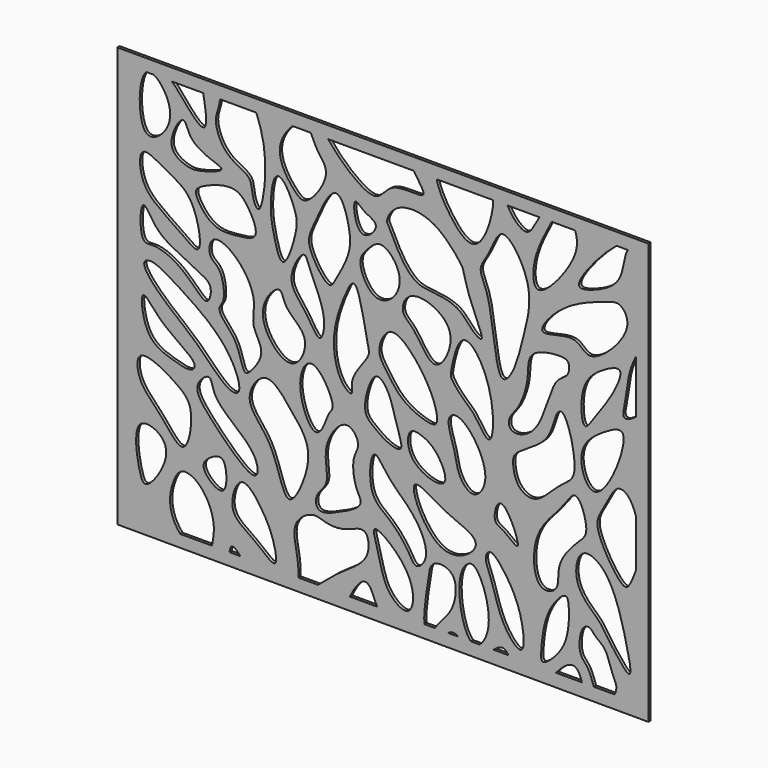
from build123d import *

# Parameters (mm, degrees)
F1_DEPTH = 3


with BuildPart() as f1:
    # F0 (on Front) → F1 (new body)
    with BuildSketch(Plane.XZ):
        with BuildLine():
            add(Edge.make_bspline(
                [(9.7901637022, -246.1338124736), (9.7588059123, -251.7433011661), (9.8231638207, -256.1141962417), (11.7309523035, -257.2440662537)],
                knots=[0.9400744919, 0.9400744919, 0.9400744919, 0.9400744919, 1, 1, 1, 1], degree=3))
            add(Edge.make_bspline(
                [(11.7309523035, -257.2440662537), (14.5146742843, -258.8926997454), (22.0720929935, -252.976389453), (29.3722832782, -246.8268878524), (30.1904138178, -246.1340725422)],
                knots=[0, 0, 0, 0, 0.0874394387, 0.0985039599, 0.0985039599, 0.0985039599, 0.0985039599], degree=3))
            Line((30.1904138178, -246.1340725422), (9.7901637022, -246.1338124736))
        make_face()
        with BuildLine():
            add(Edge.make_bspline(
                [(11.7309523035, -257.2440662537), (14.5146742843, -258.8926997454), (22.0720929935, -252.976389453), (29.3722832782, -246.8268878524), (30.1904138178, -246.1340725422)],
                knots=[0, 0, 0, 0, 0.0874394387, 0.0985039599, 0.0985039599, 0.0985039599, 0.0985039599], degree=3))
            add(Edge.make_bspline(
                [(9.7901637022, -246.1338124736), (9.7588059123, -251.7433011661), (9.8231638207, -256.1141962417), (11.7309523035, -257.2440662537)],
                knots=[0.9400744919, 0.9400744919, 0.9400744919, 0.9400744919, 1, 1, 1, 1], degree=3))
            Line((9.7901637022, -246.1338124736), (-50.3665320084, -246.1330455778))
            add(Edge.make_bspline(
                [(-50.3665320084, -246.1330455778), (-48.3303775027, -248.2458131265), (-43.1270763382, -253.7190469273), (-37.557143271, -257.1762818819), (-34.5870695785, -259.0077182933)],
                knots=[0.0807811304, 0.0807811304, 0.0807811304, 0.0807811304, 0.1240320576, 0.1830256289, 0.1830256289, 0.1830256289, 0.1830256289], degree=3))
            Line((-34.5870695785, -259.0077182933), (58.3993176905, -259.2085698625))
            add(Edge.make_bspline(
                [(63.4588769506, -246.1344966587), (61.4663237301, -250.3922527368), (59.7094369574, -254.9256346001), (58.3993176905, -259.2085698626)],
                knots=[0.6923882564, 0.6923882564, 0.6923882564, 0.6923882564, 0.7375587218, 0.7375587218, 0.7375587218, 0.7375587218], degree=3))
            Line((63.4588769506, -246.1344966587), (30.1904138178, -246.1340725422))
        make_face()
        with BuildLine():
            add(Edge.make_bspline(
                [(30.1904138178, -246.1340725422), (38.4358538211, -239.1516085003), (55.131623573, -224.2446867648), (85.9226539602, -207.4468162091), (81.6135257776, -174.2710504238), (59.1064210203, -188.0247219258), (38.7928820794, -187.8617203747), (24.9584000908, -180.3500590955), (-0.7627512557, -198.2249048598), (10.0492867768, -225.7411908763), (9.8094313103, -242.6870953938), (9.7901637022, -246.1338124736)],
                knots=[0.0985039599, 0.0985039599, 0.0985039599, 0.0985039599, 0.2100165383, 0.3296185811, 0.4228923825, 0.5125673919, 0.6050878351, 0.6821223818, 0.7806699981, 0.9032536186, 0.9400744919, 0.9400744919, 0.9400744919, 0.9400744919], degree=3))
            Line((30.1904138178, -246.1340725422), (63.4588769506, -246.1344966587))
            add(Edge.make_bspline(
                [(91.6403743178, -246.134855925), (88.9294590563, -239.927946458), (83.9082250339, -226.1808906061), (74.3017322339, -227.0352627662), (66.7290897392, -239.1465937843), (63.4588769506, -246.1344966587)],
                knots=[0.4782821954, 0.4782821954, 0.4782821954, 0.4782821954, 0.5486253717, 0.6182537078, 0.6923882564, 0.6923882564, 0.6923882564, 0.6923882564], degree=3))
            Line((91.6403743178, -246.134855925), (140.7887530913, -246.1354824834))
            add(Edge.make_bspline(
                [(150.9457230568, -187.4773949385), (146.6330961136, -190.0849035028), (145.0700738243, -202.6562319311), (141.9604717379, -222.0309323338), (140.3139450852, -237.0479527238), (140.7480163893, -245.5020574078), (140.7887530913, -246.1354824834)],
                knots=[0, 0, 0, 0, 0.1097664917, 0.2358758525, 0.3680330796, 0.378831128, 0.378831128, 0.378831128, 0.378831128], degree=3))
            add(Edge.make_bspline(
                [(151.6535557612, -246.1356209912), (152.0842457989, -245.492729905), (157.8673173196, -237.104152239), (172.5904347604, -225.4697199707), (176.6155565027, -187.0751886755), (155.7266048302, -184.5867692633), (150.9457230568, -187.4773949385)],
                knots=[0.5638155494, 0.5638155494, 0.5638155494, 0.5638155494, 0.575980752, 0.7233184576, 0.8783153223, 1, 1, 1, 1], degree=3))
            Line((151.6535557612, -246.1356209912), (165.5383993688, -246.1357979994))
            add(Edge.make_bspline(
                [(165.5383993688, -246.1357979994), (166.8916685862, -245.1374841957), (168.2456112198, -244.4708527481), (169.5520877838, -244.227617979)],
                knots=[0.9684245262, 0.9684245262, 0.9684245262, 0.9684245262, 1, 1, 1, 1], degree=3))
            add(Edge.make_bspline(
                [(169.5520877838, -244.227617979), (171.7348934141, -243.8212316434), (173.7852007903, -244.5967278838), (175.7411883681, -246.1359280677)],
                knots=[0, 0, 0, 0, 0.0527549624, 0.0527549624, 0.0527549624, 0.0527549624], degree=3))
            Line((175.7411883681, -246.1359280677), (189.226356025, -246.1360999807))
            add(Edge.make_bspline(
                [(185.325473547, -176.8171787262), (182.5084622348, -179.0124112443), (176.5500739638, -188.6532054998), (176.555339328, -219.1069042104), (184.7595727212, -242.227658134), (189.226356025, -246.1360999807)],
                knots=[0, 0, 0, 0, 0.1198377942, 0.3180430449, 0.4608531492, 0.4608531492, 0.4608531492, 0.4608531492], degree=3))
            add(Edge.make_bspline(
                [(198.0807921271, -246.1362128598), (202.4572107284, -242.8113384732), (214.294124997, -220.2269298488), (196.4537099683, -172.0993780413), (187.465245085, -175.1497036822), (185.325473547, -176.8171787262)],
                knots=[0.5460960759, 0.5460960759, 0.5460960759, 0.5460960759, 0.6687120885, 0.9089724986, 1, 1, 1, 1], degree=3))
            Line((198.0807921271, -246.1362128598), (212.7578583264, -246.1363999675))
            add(Edge.make_bspline(
                [(212.7578583264, -246.1363999675), (216.1131583124, -243.0848294513), (219.5559651959, -241.1799456168), (222.2440987825, -241.4247691631)],
                knots=[0.9445554177, 0.9445554177, 0.9445554177, 0.9445554177, 1, 1, 1, 1], degree=3))
            add(Edge.make_bspline(
                [(222.2440987825, -241.4247691631), (224.6132182636, -241.6405382885), (226.3961574475, -243.5260579096), (227.8743273651, -246.1365926768)],
                knots=[0, 0, 0, 0, 0.0488646995, 0.0488646995, 0.0488646995, 0.0488646995], degree=3))
            Line((227.8743273651, -246.1365926768), (277.7129229054, -246.1372280344))
            add(Edge.make_bspline(
                [(277.7129229054, -246.1372280344), (283.6923653133, -238.8513551932), (296.7957777997, -228.067446888), (302.7192229603, -239.3766984719), (304.4872900639, -246.1375693621)],
                knots=[0.3680159099, 0.3680159099, 0.3680159099, 0.3680159099, 0.4564824469, 0.5466627512, 0.5466627512, 0.5466627512, 0.5466627512], degree=3))
            Line((304.4872900639, -246.1375693621), (316.9620559109, -246.1377283942))
            add(Edge.make_bspline(
                [(316.9620559109, -246.1377283942), (315.1592613006, -240.7444351763), (310.8096705188, -228.164972779), (300.0346077167, -222.3203557149), (302.9818520324, -194.8007969424), (310.2238803249, -192.6842301325), (312.23320961, -193.430557847)],
                knots=[0.6529297592, 0.6529297592, 0.6529297592, 0.6529297592, 0.7271660182, 0.8177156532, 0.9357279799, 1, 1, 1, 1], degree=3))
            add(Edge.make_bspline(
                [(312.23320961, -193.430557847), (314.3987465407, -194.2349059647), (317.9201942459, -200.0632035933), (330.6257744805, -206.8171760044), (334.6111704969, -227.0036269584), (341.6905925863, -237.1679193511), (339.7554115606, -243.7170809246), (338.6080290375, -246.1380043437)],
                knots=[0, 0, 0, 0, 0.0692686033, 0.1590658267, 0.2671580117, 0.3555247119, 0.4051353819, 0.4051353819, 0.4051353819, 0.4051353819], degree=3))
            Line((338.6080290375, -246.1380043437), (360.9821200371, -246.1382895754))
            Line((360.9821200371, -246.1382895754), (360.9821200371, -124.6424126949))
            add(Edge.make_bspline(
                [(342.0082628727, -56.7098855972), (337.8376569664, -58.6143161112), (331.7078660667, -71.4640421648), (322.8482168883, -85.7041512548), (316.6274138765, -102.0127331196), (347.5547979066, -150.7207499406), (354.6205927365, -140.2264698905), (359.0749163627, -130.6088737094), (360.9821200371, -124.6424126949)],
                knots=[0, 0, 0, 0, 0.1084019294, 0.2154866103, 0.3238733132, 0.5061092667, 0.5780773791, 0.6571797703, 0.6571797703, 0.6571797703, 0.6571797703], degree=3))
            add(Edge.make_bspline(
                [(360.9821200371, -76.531337101), (359.0514846438, -70.245651789), (353.2660580691, -58.0597419764), (345.5294972833, -55.1019786386), (342.0082628727, -56.7098855972)],
                knots=[0.8351803062, 0.8351803062, 0.8351803062, 0.8351803062, 0.908476463, 1, 1, 1, 1], degree=3))
            Line((360.9821200371, -76.531337101), (360.9821200371, 15.1898744979))
            add(Edge.make_bspline(
                [(360.9821200371, 15.1898744979), (355.6565059721, 11.1423212631), (350.6052370501, 8.7464678831), (348.6705720425, 10.5318771675)],
                knots=[0.8984641801, 0.8984641801, 0.8984641801, 0.8984641801, 1, 1, 1, 1], degree=3))
            add(Edge.make_bspline(
                [(348.6705720425, 10.5318771675), (346.1789182244, 12.8313046357), (352.3475964652, 34.1049078926), (352.0242052067, 51.6807917861), (359.6520995719, 68.2783470175), (360.9821200371, 70.9079119016)],
                knots=[0, 0, 0, 0, 0.1307679171, 0.3012406905, 0.3329604649, 0.3329604649, 0.3329604649, 0.3329604649], degree=3))
            Line((360.9821200371, 70.9079119016), (360.9821200371, 165.1975970457))
            Line((360.9821200371, 165.1975970457), (352.5482071967, 165.1975970457))
            add(Edge.make_bspline(
                [(352.4027168751, 164.9963259697), (352.4506544554, 165.0640860413), (352.4991627821, 165.131172959), (352.5482071967, 165.1975970457)],
                knots=[0.5045050801, 0.5045050801, 0.5045050801, 0.5045050801, 0.5064013288, 0.5064013288, 0.5064013288, 0.5064013288], degree=3))
            add(Edge.make_bspline(
                [(301.554620266, 116.592861712), (301.9530032289, 112.4990153253), (320.233240766, 117.1712219456), (349.144625433, 132.3748423439), (347.8079865703, 158.5016457505), (352.4027168751, 164.9963259697)],
                knots=[0, 0, 0, 0, 0.1299762549, 0.3227530746, 0.5045050801, 0.5045050801, 0.5045050801, 0.5045050801], degree=3))
            add(Edge.make_bspline(
                [(340.6141401268, 165.1975970457), (323.4581870006, 151.6388907619), (300.8248964657, 124.0916189903), (301.554620266, 116.592861712)],
                knots=[0.7619206254, 0.7619206254, 0.7619206254, 0.7619206254, 1, 1, 1, 1], degree=3))
            Line((340.6141401268, 165.1975970457), (316.197607198, 165.1975970457))
            add(Edge.make_bspline(
                [(312.9373053891, 165.1975970457), (313.7379383521, 164.6227509115), (314.7385961218, 164.5574802886), (316.0388133955, 165.1217950158), (316.197607198, 165.1975970457)],
                knots=[0.3221219636, 0.3221219636, 0.3221219636, 0.3221219636, 0.3594895273, 0.3645407278, 0.3645407278, 0.3645407278, 0.3645407278], degree=3))
            Line((312.9373053891, 165.1975970457), (297.5711116065, 165.1975970457))
            add(Edge.make_bspline(
                [(297.5711116065, 165.1975970457), (299.4289483797, 159.056886812), (303.0083586173, 140.1668971596), (268.7535906867, 98.0109773184), (259.5071792603, 98.5026732087)],
                knots=[0.6614479245, 0.6614479245, 0.6614479245, 0.6614479245, 0.7737000347, 1, 1, 1, 1], degree=3))
            add(Edge.make_bspline(
                [(259.5071792603, 98.5026732087), (254.0550463277, 98.7926009691), (252.3186900207, 124.0218742831), (263.2709078544, 146.1532628497), (272.1856793908, 163.3292534028), (273.1705281061, 165.1975970457)],
                knots=[0, 0, 0, 0, 0.1334374425, 0.3281816369, 0.3520603533, 0.3520603533, 0.3520603533, 0.3520603533], degree=3))
            Line((273.1705281061, 165.1975970457), (260.5168320192, 165.1975970457))
            add(Edge.make_bspline(
                [(245.8173036575, 147.3950594664), (250.5583563735, 147.0523913273), (253.9924391368, 154.4900621523), (259.1169298408, 162.9643350938), (260.5168320192, 165.1975970457)],
                knots=[0, 0, 0, 0, 0.0827283575, 0.1116799116, 0.1116799116, 0.1116799116, 0.1116799116], degree=3))
            add(Edge.make_bspline(
                [(227.3503893477, 165.1975970457), (231.4225669247, 156.4975025172), (240.1755924408, 147.8028243236), (245.8173036575, 147.3950594664)],
                knots=[0.9015557239, 0.9015557239, 0.9015557239, 0.9015557239, 1, 1, 1, 1], degree=3))
            Line((227.3503893477, 165.1975970457), (212.3341254649, 165.1975970457))
            add(Edge.make_bspline(
                [(155.0230979919, 160.0361615419), (156.8732559449, 154.6766413761), (163.0714439049, 142.2896208272), (181.5890181301, 117.4369562013), (199.8519668676, 117.5588360405), (210.5976716303, 145.8389913841), (212.3245910057, 161.3691844962), (212.3341254649, 165.1975970457)],
                knots=[0, 0, 0, 0, 0.1072129517, 0.2385789935, 0.3255263098, 0.4690536374, 0.5179348553, 0.5179348553, 0.5179348553, 0.5179348553], degree=3))
            add(Edge.make_bspline(
                [(153.6499642193, 165.1975970457), (153.940582741, 163.4251992855), (154.4345182879, 161.7411536958), (155.0230979919, 160.0361615419)],
                knots=[0.9658929837, 0.9658929837, 0.9658929837, 0.9658929837, 1, 1, 1, 1], degree=3))
            Line((153.6499642193, 165.1975970457), (129.826022755, 165.1975970457))
            add(Edge.make_bspline(
                [(91.6477292776, 129.5943558216), (97.3979884485, 131.7922597709), (105.2485675897, 149.8823023767), (147.9146265598, 140.6352041492), (135.593177157, 155.9927611171), (130.8858030033, 163.4806066542), (129.826022755, 165.1975970457)],
                knots=[0, 0, 0, 0, 0.0856459715, 0.1836942568, 0.253366065, 0.274225406, 0.274225406, 0.274225406, 0.274225406], degree=3))
            add(Edge.make_bspline(
                [(40.8015214916, 165.1975970457), (49.0526624832, 154.4726750808), (67.6534973731, 136.8247102001), (85.8715274154, 127.3865358769), (91.6477292776, 129.5943558216)],
                knots=[0.8012274033, 0.8012274033, 0.8012274033, 0.8012274033, 0.9139676307, 1, 1, 1, 1], degree=3))
            Line((40.8015214916, 165.1975970457), (22.6455849149, 165.1975970457))
            add(Edge.make_bspline(
                [(22.6455849149, 165.1975970457), (24.6398958382, 161.6370109703), (29.5538657027, 148.2355516574), (47.0601388111, 135.1221054363), (18.7166898876, 95.5205719357), (5.0069116738, 106.1424772606), (-17.6160930997, 136.0140279301), (-2.2030845369, 159.677612741), (3.8405073166, 165.1975970457)],
                knots=[0.0698097678, 0.0698097678, 0.0698097678, 0.0698097678, 0.1481908, 0.2995346732, 0.4930544209, 0.6052153218, 0.8046207697, 0.9189939387, 0.9189939387, 0.9189939387, 0.9189939387], degree=3))
            Line((3.8405073166, 165.1975970457), (-34.0658859726, 165.1975970457))
            add(Edge.make_bspline(
                [(-71.6462448819, 165.1975970457), (-72.2969683467, 157.3510943413), (-79.7183107043, 145.6816655054), (-68.6377171634, 119.6547763879), (-53.3257447767, 110.2585347544), (-38.2399788393, 103.6005996281), (-38.614635353, 86.7659803961), (-31.1317027167, 72.1252851471), (-24.62202919, 96.8150655062), (-23.2706553709, 134.0637171072), (-30.9532538043, 157.4744689897), (-34.0658859726, 165.1975970457)],
                knots=[0.089928055, 0.089928055, 0.089928055, 0.089928055, 0.1676987467, 0.2527597183, 0.3254280955, 0.3898837418, 0.4591848219, 0.5122515839, 0.581435558, 0.6977227887, 0.7653792045, 0.7653792045, 0.7653792045, 0.7653792045], degree=3))
            Line((-71.6462448819, 165.1975970457), (-89.0812227176, 165.1975970457))
            add(Edge.make_bspline(
                [(-89.0812227176, 165.1975970457), (-86.8017226668, 153.5122763774), (-81.940175123, 120.319503587), (-107.9165107445, 149.4971925596), (-117.6975816285, 161.9199339716), (-121.8640712604, 165.1975970457)],
                knots=[0.3704020456, 0.3704020456, 0.3704020456, 0.3704020456, 0.4942900576, 0.6199661345, 0.6995310505, 0.6995310505, 0.6995310505, 0.6995310505], degree=3))
            Line((-121.8640712604, 165.1975970457), (-140.5946574464, 165.1975970457))
            add(Edge.make_bspline(
                [(-140.5946574464, 165.1975970457), (-134.9257063203, 162.2886488757), (-119.4787882332, 141.7502735529), (-125.928966429, 114.6992790111), (-144.2378376817, 104.6267474873), (-149.1714119911, 110.2871596813)],
                knots=[0.401597112, 0.401597112, 0.401597112, 0.401597112, 0.5621504349, 0.8086075159, 1, 1, 1, 1], degree=3))
            add(Edge.make_bspline(
                [(-149.1714119911, 110.2871596813), (-157.5416921129, 119.8905897092), (-157.0763635952, 158.4606170832), (-148.0610253078, 165.1975970457)],
                knots=[0, 0, 0, 0, 0.324715633, 0.324715633, 0.324715633, 0.324715633], degree=3))
            Line((-148.0610253078, 165.1975970457), (-165.7420098782, 165.1975970457))
            Line((-165.7420098782, 165.1975970457), (-165.7420098782, -246.1382895754))
            Line((-165.7420098782, -246.1382895754), (-113.0190528962, -246.1382895754))
            add(Edge.make_bspline(
                [(-111.2022027373, -188.2839649916), (-115.7367334985, -190.1385830578), (-121.4688091599, -202.2879183309), (-125.0870479005, -219.505637695), (-121.1606821222, -235.3049207758), (-114.6758142992, -244.1395123904), (-113.0190528962, -246.1382895754)],
                knots=[0, 0, 0, 0, 0.0923866418, 0.1889201522, 0.2950886497, 0.3264831601, 0.3264831601, 0.3264831601, 0.3264831601], degree=3))
            add(Edge.make_bspline(
                [(-79.9855316672, -246.1326679858), (-78.979360547, -240.8248467781), (-75.4830066636, -221.8614278802), (-89.7581656824, -192.8295221067), (-106.360277204, -186.3036228035), (-111.2022027373, -188.2839649916)],
                knots=[0.7014049055, 0.7014049055, 0.7014049055, 0.7014049055, 0.7597148887, 0.9013504895, 1, 1, 1, 1], degree=3))
            Line((-79.9855316672, -246.1326679858), (-61.7217507226, -246.132900818))
            add(Edge.make_bspline(
                [(-61.7217507226, -246.132900818), (-61.3553102235, -242.982915953), (-60.5950676776, -240.7594567784), (-59.4025216997, -240.0836497545)],
                knots=[0.9519600349, 0.9519600349, 0.9519600349, 0.9519600349, 1, 1, 1, 1], degree=3))
            add(Edge.make_bspline(
                [(-59.4025216997, -240.0836497545), (-57.397207753, -238.9472531079), (-54.1695224407, -242.186962532), (-50.3665320084, -246.1330455778)],
                knots=[0, 0, 0, 0, 0.0807811304, 0.0807811304, 0.0807811304, 0.0807811304], degree=3))
            Line((-50.3665320084, -246.1330455778), (9.7901637022, -246.1338124736))
        make_face()
        with BuildLine():
            add(Edge.make_bspline(
                [(-49.0425825119, -177.9240220785), (-42.8470364952, -175.9658380857), (-26.747837749, -196.6289989175), (-15.6036590183, -218.4973309131), (-10.2543517306, -250.6961493178), (-37.5967274964, -223.2187291122), (-65.5230366459, -210.84902308), (-55.5631052255, -179.9849192405), (-49.0425825119, -177.9240220785)],
                knots=[0, 0, 0, 0, 0.163821842, 0.3437585205, 0.4833218477, 0.6484554387, 0.8275851654, 1, 1, 1, 1], degree=3))
        make_face(mode=Mode.SUBTRACT)
        with BuildLine():
            add(Edge.make_bspline(
                [(-154.7139436007, -159.2761427164), (-162.0673137426, -166.5822235647), (-156.2899293947, -203.4468910848), (-148.775531084, -218.1461415178), (-125.5891043797, -187.0420821525), (-127.5237587016, -161.4356635882), (-149.5291516341, -154.124693985), (-154.7139436007, -159.2761427164)],
                knots=[0, 0, 0, 0, 0.2661661973, 0.3945228903, 0.6168433641, 0.8123287235, 1, 1, 1, 1], degree=3))
        make_face(mode=Mode.SUBTRACT)
        with BuildLine():
            add(Edge.make_bspline(
                [(-154.7139436007, -117.8363934159), (-150.3330004414, -128.1604054443), (-133.7235727782, -140.5181794193), (-107.025270693, -181.4076993717), (-97.9114632331, -127.5386921075), (-112.5996499207, -110.9999080575), (-160.1993723872, -84.4868963537), (-158.1885838415, -109.6481503056), (-154.7139436007, -117.8363934159)],
                knots=[0, 0, 0, 0, 0.1762482162, 0.3424839636, 0.5175769137, 0.6707372224, 0.8602129445, 1, 1, 1, 1], degree=3))
        make_face(mode=Mode.SUBTRACT)
        with BuildLine():
            add(Edge.make_bspline(
                [(-83.1116363406, -167.107462883), (-86.8950146982, -170.0166810192), (-94.1015318841, -178.4470759392), (-64.2507972163, -203.6432671878), (-64.3495703263, -169.2194988193), (-70.9241249433, -160.0006980719), (-79.3594135294, -164.2222017165), (-83.1116363406, -167.107462883)],
                knots=[0, 0, 0, 0, 0.1793282299, 0.4240380764, 0.6648174361, 0.8221485109, 1, 1, 1, 1], degree=3))
        make_face(mode=Mode.SUBTRACT)
        with BuildLine():
            add(Edge.make_bspline(
                [(-94.6263149381, -103.3324822783), (-97.3351273693, -111.3066536379), (-82.1513836519, -130.6274937722), (-30.5261311673, -182.3501636577), (-32.2249762364, -141.5247921608), (-80.830203768, -114.8528230357), (-79.6288248503, -86.5475214013), (-92.7324826989, -97.7574403792), (-94.6263149381, -103.3324822783)],
                knots=[0, 0, 0, 0, 0.1696352952, 0.3986729263, 0.5292755047, 0.7562551812, 0.8814016108, 1, 1, 1, 1], degree=3))
        make_face(mode=Mode.SUBTRACT)
        with BuildLine():
            add(Edge.make_bspline(
                [(-151.437535882, -40.0536358356), (-149.2210512947, -38.4603234546), (-137.7795959471, -54.3524178919), (-118.0480813781, -69.3715854838), (-94.7919748909, -84.598481614), (-101.4264509751, -94.8120633896), (-122.7162799821, -88.8718402019), (-150.44874113, -79.5390002198), (-154.5821508584, -42.3141315793), (-151.437535882, -40.0536358356)],
                knots=[0, 0, 0, 0, 0.1233388014, 0.2925025537, 0.4419871436, 0.5200136835, 0.6563686945, 0.8250143294, 1, 1, 1, 1], degree=3))
        make_face(mode=Mode.SUBTRACT)
        with BuildLine():
            add(Edge.make_bspline(
                [(-150.5026966333, -11.0736070201), (-150.4893487051, -17.3355469245), (-126.2152665406, -42.6351071505), (-94.7569613857, -64.5684509849), (-65.3041487641, -99.3539826394), (-46.6543602503, -98.6276226274), (-62.6024893437, -54.8362913711), (-110.5945621284, -22.9231924262), (-143.0495610241, -2.8415781502), (-150.5087707517, -8.224043874), (-150.5026966333, -11.0736070201)],
                knots=[0, 0, 0, 0, 0.1322321478, 0.2823248202, 0.4289628952, 0.4972210274, 0.6304299889, 0.8086347478, 0.939826338, 1, 1, 1, 1], degree=3))
        make_face(mode=Mode.SUBTRACT)
        with BuildLine():
            add(Edge.make_bspline(
                [(0, -177.4109601974), (5.8200221993, -178.1370236931), (21.2026976084, -145.2132493719), (20.6495023203, -117.3443166746), (1.0015963147, -94.1253142853), (-24.1127550851, -63.1248739152), (-51.1629892185, -103.5894306607), (-14.293252374, -127.6052780443), (-6.8005060178, -176.5625786961), (0, -177.4109601974)],
                knots=[0, 0, 0, 0, 0.1427258357, 0.2751074907, 0.4104542502, 0.5445432786, 0.675497511, 0.8332295185, 1, 1, 1, 1], degree=3))
        make_face(mode=Mode.SUBTRACT)
        with BuildLine():
            add(Edge.make_bspline(
                [(29.0527436882, -165.0769263506), (31.2395066331, -159.5630187032), (44.9159701153, -150.1849526604), (31.4570289031, -118.0637373663), (59.2891467403, -79.8804512916), (75.8000423543, -104.7237414977), (64.7835769051, -116.4842560456), (67.9701329048, -144.8221419535), (79.7959889027, -159.1493961431), (53.5033760291, -172.0515429332), (28.835559846, -182.3442693433), (27.2907319165, -169.5198268512), (29.0527436882, -165.0769263506)],
                knots=[0, 0, 0, 0, 0.0933625362, 0.2163559826, 0.3440104059, 0.4348205419, 0.5177258055, 0.6310963589, 0.7117318364, 0.821188626, 0.9247719611, 1, 1, 1, 1], degree=3))
        make_face(mode=Mode.SUBTRACT)
        with BuildLine():
            add(Edge.make_bspline(
                [(24.7797649354, -46.1300946772), (33.4841423853, -48.1610374633), (49.9295556285, -77.7408917815), (41.0382183293, -84.223270109), (37.2344758871, -98.5719609378), (25.0455020105, -115.9992902392), (4.5933329876, -68.737967041), (17.5128248481, -44.4345409593), (24.7797649354, -46.1300946772)],
                knots=[0, 0, 0, 0, 0.216780114, 0.3243111701, 0.4642219083, 0.5877696991, 0.8190188661, 1, 1, 1, 1], degree=3))
        make_face(mode=Mode.SUBTRACT)
        with BuildLine():
            add(Edge.make_bspline(
                [(80.4027318954, -74.1752907634), (82.0467210946, -78.0943267376), (89.229057935, -83.1695231565), (100.5726733877, -92.4164954968), (121.2433396864, -98.0621788598), (111.0017186855, -72.9307433961), (106.2914892853, -47.8955258557), (90.5010452837, -28.504632203), (79.7990264357, -53.3568625242), (78.2222110363, -68.9772397701), (80.4027318954, -74.1752907634)],
                knots=[0, 0, 0, 0, 0.102251427, 0.2199368704, 0.3280782412, 0.4554437385, 0.6155828309, 0.7332437765, 0.8643778381, 1, 1, 1, 1], degree=3))
        make_face(mode=Mode.SUBTRACT)
        with BuildLine():
            add(Edge.make_bspline(
                [(89.410841465, -175.7564544678), (86.6030560203, -177.2233677412), (94.366061844, -197.815945156), (98.8409064083, -228.734502778), (123.7839973339, -245.6969403956), (131.9750770063, -225.5342598057), (121.9674910588, -195.3771845413), (93.1158460088, -173.8207936239), (89.410841465, -175.7564544678)],
                knots=[0, 0, 0, 0, 0.1442767921, 0.3405895945, 0.4935831484, 0.6164220744, 0.809620008, 1, 1, 1, 1], degree=3))
        make_face(mode=Mode.SUBTRACT)
        with BuildLine():
            add(Edge.make_bspline(
                [(204.7077417374, -163.8956665993), (204.1523225453, -168.6485935078), (211.6683604624, -182.3062631169), (219.8238730584, -220.7434793935), (247.1471601877, -247.7798983258), (242.2585468756, -201.0883152829), (226.7729628555, -174.0459785633), (209.8460474977, -153.4490082691), (205.0653686655, -160.8353210545), (204.7077417374, -163.8956665993)],
                knots=[0, 0, 0, 0, 0.1236765591, 0.3143041835, 0.4507721866, 0.6117599636, 0.7901366256, 0.9203663313, 1, 1, 1, 1], degree=3))
        make_face(mode=Mode.SUBTRACT)
        with BuildLine():
            add(Edge.make_bspline(
                [(263.7775242329, -240.5017912388), (266.2082045074, -241.3172040158), (278.8113733746, -230.5387872285), (291.0252753674, -211.4965624071), (291.8551974369, -179.5938069576), (287.5889582541, -168.4423483181), (266.3406562061, -191.4777978965), (262.3643964417, -225.5266234953), (261.613343229, -239.775780146), (263.7775242329, -240.5017912388)],
                knots=[0, 0, 0, 0, 0.1230988977, 0.2820872387, 0.4589053959, 0.5387575037, 0.6938434852, 0.8903976394, 1, 1, 1, 1], degree=3))
        make_face(mode=Mode.SUBTRACT)
        with BuildLine():
            add(Edge.make_bspline(
                [(88.678278029, -107.6285466552), (91.9390645239, -105.9309566943), (103.37699785, -127.335172652), (131.0999306085, -147.0863165568), (148.3542447523, -183.2261837364), (131.5732441289, -200.1687303011), (124.5569320843, -184.0548745939), (105.564771734, -160.4088417201), (81.2425974722, -148.3974638869), (84.4177193629, -109.8466255238), (88.678278029, -107.6285466552)],
                knots=[0, 0, 0, 0, 0.1102741842, 0.2642143755, 0.411244528, 0.504785479, 0.5914271891, 0.7272813755, 0.8559152426, 1, 1, 1, 1], degree=3))
        make_face(mode=Mode.SUBTRACT)
        with BuildLine():
            add(Edge.make_bspline(
                [(130.4340958595, -122.2797185183), (133.0400681692, -117.8271601762), (154.9141954368, -132.3650170442), (174.6052962396, -141.4299827917), (184.8133512468, -144.7470659296), (203.4744474996, -157.4013365851), (154.8156762099, -192.0919576276), (126.3803245372, -129.2059829497), (130.4340958595, -122.2797185183)],
                knots=[0, 0, 0, 0, 0.1600323205, 0.3226553408, 0.4319117618, 0.5546081218, 0.7510585861, 1, 1, 1, 1], degree=3))
        make_face(mode=Mode.SUBTRACT)
        with BuildLine():
            add(Edge.make_bspline(
                [(214.1752690077, -126.3125836849), (213.0041878255, -120.7514142857), (219.8665971717, -92.0211380051), (247.2077011259, -156.7016947172), (223.3830926025, -131.5769554034), (215.1725210623, -131.0482823655), (214.1752690077, -126.3125836849)],
                knots=[0, 0, 0, 0, 0.2354488004, 0.5758462886, 0.7994999804, 1, 1, 1, 1], degree=3))
        make_face(mode=Mode.SUBTRACT)
        with BuildLine():
            add(Edge.make_bspline(
                [(126.4401078224, -74.6891573071), (122.5239643988, -78.7963365946), (122.1914860804, -105.5016182127), (171.8867005439, -120.2022014193), (154.5217244599, -82.3185468825), (138.6629526756, -74.0680619172), (128.9665956425, -72.0394232902), (126.4401078224, -74.6891573071)],
                knots=[0, 0, 0, 0, 0.2145358952, 0.4572378776, 0.6719930307, 0.8615928306, 1, 1, 1, 1], degree=3))
        make_face(mode=Mode.SUBTRACT)
        with BuildLine():
            add(Edge.make_bspline(
                [(166.3480997086, -50.0724948943), (165.339349991, -53.8293485495), (167.8059829942, -64.5023735653), (172.8796792164, -77.7862206967), (175.1067187168, -98.9759395974), (192.7650047576, -117.4716066646), (211.7732201054, -90.28459381), (188.8626985545, -50.1715455029), (171.8555726807, -42.495848002), (167.0896117461, -47.3109058102), (166.3480997086, -50.0724948943)],
                knots=[0, 0, 0, 0, 0.1072274123, 0.2184521607, 0.3534504855, 0.4775216841, 0.6138949518, 0.806442624, 0.9211792424, 1, 1, 1, 1], degree=3))
        make_face(mode=Mode.SUBTRACT)
        with BuildLine():
            add(Edge.make_bspline(
                [(298.4280288219, -77.6777416468), (294.3040478163, -76.2921197484), (285.3245136432, -92.9330899627), (266.9607307519, -109.5939483237), (254.2974671212, -132.5074819859), (253.9787997513, -162.4284662391), (264.0055531453, -177.0898088384), (282.7198889127, -169.7764116334), (276.3853521731, -144.0342812686), (301.8707693717, -117.4401451098), (313.0906701859, -107.3213697907), (303.6815574574, -79.4428817652), (298.4280288219, -77.6777416468)],
                knots=[0, 0, 0, 0, 0.089039436, 0.1991282231, 0.3063955203, 0.4206241499, 0.5006279828, 0.5781437498, 0.679347374, 0.8034575627, 0.8865728949, 1, 1, 1, 1], degree=3))
        make_face(mode=Mode.SUBTRACT)
        with BuildLine():
            add(Edge.make_bspline(
                [(320.2433586121, -182.1674406528), (315.0293316685, -177.2312605891), (294.1076481921, -160.5979135941), (301.2426859067, -119.5148667501), (335.3720060402, -135.3617989296), (350.0969142683, -190.8118410895), (360.1255769026, -238.3022753521), (326.6233242913, -190.0170173632), (323.5883525267, -185.3341853692), (320.2433586121, -182.1674406528)],
                knots=[0, 0, 0, 0, 0.1448937229, 0.2850223124, 0.4100184393, 0.6163278528, 0.7466596125, 0.9070452403, 1, 1, 1, 1], degree=3))
        make_face(mode=Mode.SUBTRACT)
        with BuildLine():
            add(Edge.make_bspline(
                [(236.7578595877, -58.3544187248), (233.4174400822, -61.5484116014), (232.2154075405, -68.4015899654), (236.0209966684, -89.5785470863), (257.8189356159, -99.9048926577), (279.7234921928, -72.2889373982), (300.9871564905, -62.6496735389), (294.0883347349, -29.2864091892), (292.9212875683, -23.6663982251), (285.4334244258, -1.6793656627), (275.5688921703, -10.0688717682), (272.9732415071, -39.5210960893), (243.000607579, -52.3853203579), (236.7578595877, -58.3544187248)],
                knots=[0, 0, 0, 0, 0.067514333, 0.1583364668, 0.2452279255, 0.3606221189, 0.4560086657, 0.5648975457, 0.6243667374, 0.7119562791, 0.7653898758, 0.8738257378, 1, 1, 1, 1], degree=3))
        make_face(mode=Mode.SUBTRACT)
        with BuildLine():
            add(Edge.make_bspline(
                [(347.3724424839, -5.4615912959), (345.2195292571, 0.3874205669), (324.6361905848, -10.2574458769), (295.0940784516, -32.7534033867), (320.6048718538, -95.3127561624), (351.3976862076, -16.3973308311), (347.3724424839, -5.4615912959)],
                knots=[0, 0, 0, 0, 0.1796549949, 0.4336000666, 0.6641039074, 1, 1, 1, 1], degree=3))
        make_face(mode=Mode.SUBTRACT)
        with BuildLine():
            add(Edge.make_bspline(
                [(-151.6059488058, 11.3128526136), (-149.3798551947, 7.3893555465), (-139.9648752587, 10.7958943555), (-114.7217519914, 1.7312201287), (-95.7975455291, -17.9277231696), (-83.6696896897, -28.5262345852), (-78.2790532967, -6.6581852782), (-95.1563757028, -0.0282237454), (-113.2676165813, 10.4175834954), (-138.4016960326, 21.081615298), (-154.6352779406, 57.3869444624), (-155.3702896301, 17.9475152846), (-151.6059488058, 11.3128526136)],
                knots=[0, 0, 0, 0, 0.0730757962, 0.1867694464, 0.3070742426, 0.3783772842, 0.4629846991, 0.5508638376, 0.6533204988, 0.775049667, 0.876428286, 1, 1, 1, 1], degree=3))
        make_face(mode=Mode.SUBTRACT)
        with BuildLine():
            add(Edge.make_bspline(
                [(-81.8166136742, 19.182773307), (-80.2539508362, 15.2762278257), (-72.2576816477, 12.0668172679), (-67.3849261888, -4.1070812468), (-67.2941254387, -19.2564305023), (-72.7816705771, -24.5718765297), (-71.8239761949, -32.9791739862), (-56.2985866061, -47.1317402623), (-50.6057788248, -63.5886148545), (-46.1626891661, -80.6240320269), (-35.4632495111, -68.8237000417), (-23.9760656941, -50.7896670972), (-40.926238467, -30.6456193094), (-31.8285389908, -6.1936935271), (-52.5071219439, 28.66902473), (-81.3960867178, 41.1367863034), (-83.6324593679, 23.722257844), (-81.8166136742, 19.182773307)],
                knots=[0, 0, 0, 0, 0.0554253192, 0.1213375229, 0.183982949, 0.2258764665, 0.2687988252, 0.3421561502, 0.414303499, 0.4713818425, 0.5252824466, 0.598253573, 0.6747043116, 0.7540965781, 0.856847305, 0.9355946627, 1, 1, 1, 1], degree=3))
        make_face(mode=Mode.SUBTRACT)
        with BuildLine():
            add(Edge.make_bspline(
                [(-151.6059488058, 91.0613387823), (-156.3018802011, 87.9376267161), (-154.5932795614, 60.0824020216), (-132.1660266959, 42.7520124236), (-108.1155284413, 26.5091463612), (-88.0162041009, 12.5114862152), (-97.6934696398, 69.1421543081), (-125.5860772804, 79.203447857), (-146.9991068358, 94.1257889706), (-151.6059488058, 91.0613387823)],
                knots=[0, 0, 0, 0, 0.1385770712, 0.2860835573, 0.437431789, 0.5332739116, 0.7066296756, 0.8640519604, 1, 1, 1, 1], degree=3))
        make_face(mode=Mode.SUBTRACT)
        with BuildLine():
            add(Edge.make_bspline(
                [(-96.4927151799, 70.5945715308), (-97.1445705975, 73.9099047181), (-93.342132613, 79.411279165), (-59.7692292335, 92.3242145804), (-43.70754478, 80.4647991692), (-27.5101979566, 48.7438930347), (-54.4682863564, 46.0440860026), (-80.260468959, 42.9340898534), (-95.3040067056, 64.5488065515), (-96.4927151799, 70.5945715308)],
                knots=[0, 0, 0, 0, 0.0874891474, 0.2604537834, 0.3954177852, 0.5522603277, 0.6843607147, 0.8404568128, 1, 1, 1, 1], degree=3))
        make_face(mode=Mode.SUBTRACT)
        with BuildLine():
            add(Edge.make_bspline(
                [(-9.9380407482, 10.7881957665), (-6.7813190381, 10.1077015842), (-5.4658670019, -6.3470134411), (25.1686083414, -21.461862659), (5.4495916634, -64.1163711382), (-26.0876361713, -35.228723955), (-30.0263720386, -5.6048144321), (-13.6822825981, 11.5953416065), (-9.9380407482, 10.7881957665)],
                knots=[0, 0, 0, 0, 0.1274224494, 0.3081304632, 0.4854092391, 0.6670888266, 0.8488620438, 1, 1, 1, 1], degree=3))
        make_face(mode=Mode.SUBTRACT)
        with BuildLine():
            add(Edge.make_bspline(
                [(2.6538253296, 26.0033663362), (2.3151433995, 15.5438583824), (17.2018057872, 3.4710662656), (32.7212863347, -29.9778019191), (40.5384214792, 4.2242588378), (21.3537545083, 37.2288907015), (16.2956704412, 59.5009399812), (2.982959619, 36.1680146734), (2.6538253296, 26.0033663362)],
                knots=[0, 0, 0, 0, 0.1803229441, 0.3437858765, 0.4920085246, 0.7092333915, 0.8247604647, 1, 1, 1, 1], degree=3))
        make_face(mode=Mode.SUBTRACT)
        with BuildLine():
            add(Edge.make_bspline(
                [(64.977876842, -59.6852749586), (66.2361939965, -58.7368362536), (63.2739006632, -48.4186761859), (73.7211659214, -31.7886047692), (84.8496963746, -18.0831281773), (80.8041900806, -8.3247897289), (71.062749399, 55.3337215464), (56.0273671679, 24.7276679779), (42.3579839277, -14.217901354), (51.5343768524, -52.9717929217), (63.62868684, -60.7022077833), (64.977876842, -59.6852749586)],
                knots=[0, 0, 0, 0, 0.0721860763, 0.1795323063, 0.272600743, 0.3551265897, 0.5210300759, 0.6153739733, 0.775255838, 0.9226008069, 1, 1, 1, 1], degree=3))
        make_face(mode=Mode.SUBTRACT)
        with BuildLine():
            add(Edge.make_bspline(
                [(-13.6106684804, 113.0971089005), (-17.3536783556, 109.1051634453), (-20.0521528462, 82.7510022911), (-16.9712706634, 63.4749859655), (-6.5163382712, 22.0726986217), (9.0030436257, 71.2377939208), (8.2893255141, 85.9866870156), (-4.3752347398, 114.1067847683), (-11.7533398007, 115.0779625528), (-13.6106684804, 113.0971089005)],
                knots=[0, 0, 0, 0, 0.1576687651, 0.3114270769, 0.4578920584, 0.6300857383, 0.7636739788, 0.9217627714, 1, 1, 1, 1], degree=3))
        make_face(mode=Mode.SUBTRACT)
        with BuildLine():
            add(Edge.make_bspline(
                [(96.0435047746, 86.339391768), (103.1987963098, 85.4938709718), (120.4820448664, 66.1768986969), (110.0597110789, 38.8668986576), (86.1212683542, 31.462303303), (69.4453048223, 64.3919784427), (81.3728365866, 77.543646222), (90.5060363027, 86.9937389358), (96.0435047746, 86.339391768)],
                knots=[0, 0, 0, 0, 0.185945068, 0.3658273325, 0.5193699216, 0.7118731223, 0.8560974146, 1, 1, 1, 1], degree=3))
        make_face(mode=Mode.SUBTRACT)
        with BuildLine():
            add(Edge.make_bspline(
                [(41.4787493646, 32.2992987931), (44.4610064892, 31.5099787715), (48.9579424473, 39.9648753842), (63.2361865428, 65.2028399617), (65.0177630652, 87.4080087045), (49.3669893393, 137.4887382037), (24.436733287, 78.7574808167), (16.6349449733, 61.8182137954), (35.8507143524, 33.7888821965), (41.4787493646, 32.2992987931)],
                knots=[0, 0, 0, 0, 0.0841023715, 0.2317978, 0.373311161, 0.526940071, 0.7078208309, 0.8412842785, 1, 1, 1, 1], degree=3))
        make_face(mode=Mode.SUBTRACT)
        with BuildLine():
            add(Edge.make_bspline(
                [(68.5957670212, 116.8998628855), (66.2331811818, 113.465084212), (71.317603931, 77.1096017408), (98.1063392618, 104.4141342221), (77.8795885261, 109.2937452476), (70.0835826416, 119.0628815906), (68.5957670212, 116.8998628855)],
                knots=[0, 0, 0, 0, 0.3125602194, 0.5662484428, 0.8031682198, 1, 1, 1, 1], degree=3))
        make_face(mode=Mode.SUBTRACT)
        with BuildLine():
            add(Edge.make_bspline(
                [(-110.2612689137, 133.6332410574), (-107.1312429209, 134.1172792489), (-104.6723189726, 116.9383319977), (-81.4593189552, 106.7765096169), (-62.8000206963, 101.191714982), (-94.0492118994, 91.7549732702), (-105.3203248285, 91.567224592), (-130.6748851893, 103.1490945692), (-114.6979323877, 132.9471398655), (-110.2612689137, 133.6332410574)],
                knots=[0, 0, 0, 0, 0.1233900067, 0.2941292951, 0.3976579198, 0.5538517634, 0.6770599912, 0.8251005145, 1, 1, 1, 1], degree=3))
        make_face(mode=Mode.SUBTRACT)
        with BuildLine():
            add(Edge.make_bspline(
                [(93.9448624849, -11.2475734204), (94.1278993049, -17.2644657594), (101.8381113176, -27.1241663584), (115.9224474584, -49.535334633), (141.0694424753, -60.1230039536), (158.0816026784, -61.6077061269), (147.7701853264, -24.1185570492), (116.7356639246, 11.7893859225), (100.2056974252, 10.1821816969), (93.7461989847, -4.716991799), (93.9448624849, -11.2475734204)],
                knots=[0, 0, 0, 0, 0.1087133962, 0.242913351, 0.3795882684, 0.4632698454, 0.6105469108, 0.7912206362, 0.88200525, 1, 1, 1, 1], degree=3))
        make_face(mode=Mode.SUBTRACT)
        with BuildLine():
            add(Edge.make_bspline(
                [(119.1285923123, 31.2499795109), (120.7007307114, 27.3869298901), (130.6150842447, 22.2521293259), (146.4274773894, -8.778905633), (162.169774604, -1.3784468867), (176.5470944722, 36.5831179405), (135.4844370513, 55.8658118314), (119.106393937, 45.6683769094), (117.6756910273, 34.8200403667), (119.1285923123, 31.2499795109)],
                knots=[0, 0, 0, 0, 0.1196303335, 0.2923526412, 0.3984582721, 0.5767747836, 0.7636650197, 0.889442898, 1, 1, 1, 1], degree=3))
        make_face(mode=Mode.SUBTRACT)
        with BuildLine():
            add(Edge.make_bspline(
                [(168.9713895321, -3.377659712), (168.1060921189, -8.064681166), (167.6124147615, -12.5465270994), (183.3316471979, -29.5653679077), (193.2422372021, -36.1801700035), (212.8266158799, -71.605492816), (214.677883903, -5.0939156674), (179.0252970778, 45.5776248689), (170.5860033675, 5.3681536596), (168.9713895321, -3.377659712)],
                knots=[0, 0, 0, 0, 0.0869055743, 0.2135571138, 0.325100517, 0.456335158, 0.6515880723, 0.8378373257, 1, 1, 1, 1], degree=3))
        make_face(mode=Mode.SUBTRACT)
        with BuildLine():
            add(Edge.make_bspline(
                [(102.0269095898, 110.7517033815), (101.8845505897, 108.9978514734), (104.3182580802, 105.9998183069), (113.773076348, 83.6257896277), (130.9625399321, 61.7273462338), (150.5544198867, 60.7675510189), (177.8267584769, 56.6577600205), (188.4785154174, 39.1950854994), (206.7514712946, 28.265750184), (186.7792813909, 66.0303940277), (182.0138534681, 89.3487135391), (179.1456003251, 96.4421033086), (155.5721435857, 124.7025455987), (126.7406069999, 131.4253222939), (108.2210639083, 124.9846066909), (102.2648685334, 113.6833392264), (102.0269095898, 110.7517033815)],
                knots=[0, 0, 0, 0, 0.0354384286, 0.1138109413, 0.1974466535, 0.2670273974, 0.3486534731, 0.4230784827, 0.4739842312, 0.5653227888, 0.6468875656, 0.6902661037, 0.784726632, 0.8718426836, 0.9407632041, 1, 1, 1, 1], degree=3))
        make_face(mode=Mode.SUBTRACT)
        with BuildLine():
            add(Edge.make_bspline(
                [(199.3973851204, 98.3396396041), (198.848213927, 92.4270706522), (211.5968112522, 77.3267534104), (215.1317821538, -6.1599945324), (235.2288276804, 14.6731204088), (244.4678117802, 55.0809885143), (256.5428475677, 98.7080483068), (220.9107562756, 152.0583844908), (209.9593438365, 115.0378808396), (199.8906017044, 103.6497816806), (199.3973851204, 98.3396396041)],
                knots=[0, 0, 0, 0, 0.1092735533, 0.2884414678, 0.3634463676, 0.5038416967, 0.6541785058, 0.7954926893, 0.9018602408, 1, 1, 1, 1], degree=3))
        make_face(mode=Mode.SUBTRACT)
        with BuildLine():
            add(Edge.make_bspline(
                [(229.2910963297, -29.2877070606), (230.6268804871, -25.1057119101), (239.2174833951, -17.8360603857), (250.5745374481, 12.6480552709), (246.3829498532, 41.1265334839), (280.5693691353, 46.1770480796), (292.3790592317, 43.8180071094), (291.0414757934, 27.5471711656), (272.6132767521, 23.8079080093), (263.3887663098, -35.9874887758), (229.0947824847, -43.9425428285), (228.1755967932, -32.7800479646), (229.2910963297, -29.2877070606)],
                knots=[0, 0, 0, 0, 0.0830307761, 0.206654475, 0.3141615313, 0.4314351977, 0.5005913117, 0.5741696103, 0.6593825237, 0.8229608152, 0.9306618575, 1, 1, 1, 1], degree=3))
        make_face(mode=Mode.SUBTRACT)
        with BuildLine():
            add(Edge.make_bspline(
                [(307.5106739998, -10.3224636987), (309.928946227, -11.6041654187), (319.0074173575, 3.3538652013), (336.8254872461, 25.8603572924), (350.4728021085, 59.0875195768), (322.0624389815, 45.6116345854), (301.5846088091, 26.9292526758), (303.8987727281, -8.4081299772), (307.5106739998, -10.3224636987)],
                knots=[0, 0, 0, 0, 0.1250117247, 0.3226313923, 0.4827733354, 0.6272919009, 0.8132840454, 1, 1, 1, 1], degree=3))
        make_face(mode=Mode.SUBTRACT)
        with BuildLine():
            add(Edge.make_bspline(
                [(264.1555964947, 61.5701451898), (260.1040888838, 64.4228876049), (284.7004201034, 96.8131392033), (330.8939783726, 110.2746186075), (344.220483289, 115.0905165946), (362.0200718931, 92.1770926081), (311.0917491263, 42.2063573027), (300.2872115268, 73.3191877519), (268.0783110581, 58.8080883723), (264.1555964947, 61.5701451898)],
                knots=[0, 0, 0, 0, 0.1521873802, 0.3410124096, 0.4296576036, 0.545184937, 0.7364935442, 0.8526504921, 1, 1, 1, 1], degree=3))
        make_face(mode=Mode.SUBTRACT)
        with BuildLine():
            Line((91.6403743178, -246.134855925), (63.4588769506, -246.1344966587))
            add(Edge.make_bspline(
                [(63.4588769506, -246.1344966587), (61.4663237301, -250.3922527368), (59.7094369574, -254.9256346001), (58.3993176905, -259.2085698626)],
                knots=[0.6923882564, 0.6923882564, 0.6923882564, 0.6923882564, 0.7375587218, 0.7375587218, 0.7375587218, 0.7375587218], degree=3))
            Line((58.3993176905, -259.2085698625), (115.74990898, -259.3324477397))
            add(Edge.make_bspline(
                [(115.74990898, -259.3324477397), (114.7327819445, -258.5603084657), (109.1558708328, -255.5894772217), (99.7018352267, -262.6845742087), (93.900478669, -251.3095890834), (91.6403743178, -246.134855925)],
                knots=[0.3160476927, 0.3160476927, 0.3160476927, 0.3160476927, 0.3359539089, 0.4196367183, 0.4782821954, 0.4782821954, 0.4782821954, 0.4782821954], degree=3))
        make_face()
        with BuildLine():
            add(Edge.make_bspline(
                [(-50.3665320084, -246.1330455778), (-48.3303775027, -248.2458131265), (-43.1270763382, -253.7190469273), (-37.557143271, -257.1762818819), (-34.5870695785, -259.0077182933)],
                knots=[0.0807811304, 0.0807811304, 0.0807811304, 0.0807811304, 0.1240320576, 0.1830256289, 0.1830256289, 0.1830256289, 0.1830256289], degree=3))
            Line((-50.3665320084, -246.1330455778), (-61.7217507226, -246.132900818))
            add(Edge.make_bspline(
                [(-61.5644227254, -258.9494469283), (-62.0525434962, -254.1119730658), (-62.1216684962, -249.5706620299), (-61.7217507226, -246.132900818)],
                knots=[0.8995312341, 0.8995312341, 0.8995312341, 0.8995312341, 0.9519600349, 0.9519600349, 0.9519600349, 0.9519600349], degree=3))
            Line((-61.5644227254, -258.9494469283), (-34.5870695785, -259.0077182933))
        make_face()
        with BuildLine():
            Line((140.7887530913, -246.1354824834), (91.6403743178, -246.134855925))
            add(Edge.make_bspline(
                [(115.74990898, -259.3324477397), (114.7327819445, -258.5603084657), (109.1558708328, -255.5894772217), (99.7018352267, -262.6845742087), (93.900478669, -251.3095890834), (91.6403743178, -246.134855925)],
                knots=[0.3160476927, 0.3160476927, 0.3160476927, 0.3160476927, 0.3359539089, 0.4196367183, 0.4782821954, 0.4782821954, 0.4782821954, 0.4782821954], degree=3))
            Line((115.74990898, -259.3324477397), (155.658727837, -259.4186512059))
            add(Edge.make_bspline(
                [(155.658727837, -259.4186512059), (158.3429544566, -253.7948167009), (161.9382939589, -248.7916146541), (165.5383993688, -246.1357979994)],
                knots=[0.884424216, 0.884424216, 0.884424216, 0.884424216, 0.9684245262, 0.9684245262, 0.9684245262, 0.9684245262], degree=3))
            Line((165.5383993688, -246.1357979994), (151.6535557612, -246.1356209912))
            add(Edge.make_bspline(
                [(140.7887530913, -246.1354824834), (141.1201264898, -251.2880895808), (142.9257797751, -261.4216450335), (148.2141995278, -251.2695485747), (151.6535557612, -246.1356209912)],
                knots=[0.378831128, 0.378831128, 0.378831128, 0.378831128, 0.4666680373, 0.5638155494, 0.5638155494, 0.5638155494, 0.5638155494], degree=3))
        make_face()
        with BuildLine():
            add(Edge.make_bspline(
                [(-61.5644227254, -258.9494469283), (-62.0525434962, -254.1119730658), (-62.1216684962, -249.5706620299), (-61.7217507226, -246.132900818)],
                knots=[0.8995312341, 0.8995312341, 0.8995312341, 0.8995312341, 0.9519600349, 0.9519600349, 0.9519600349, 0.9519600349], degree=3))
            Line((-61.7217507226, -246.132900818), (-79.9855316672, -246.1326679858))
            add(Edge.make_bspline(
                [(-81.8255405816, -258.9056827017), (-81.6630893988, -254.875813543), (-80.8290432554, -250.5824167481), (-79.9855316672, -246.1326679858)],
                knots=[0.6525214248, 0.6525214248, 0.6525214248, 0.6525214248, 0.7014049055, 0.7014049055, 0.7014049055, 0.7014049055], degree=3))
            Line((-81.8255405816, -258.9056827017), (-61.5644227254, -258.9494469283))
        make_face()
        with BuildLine():
            Line((151.6535557612, -246.1356209912), (140.7887530913, -246.1354824834))
            add(Edge.make_bspline(
                [(140.7887530913, -246.1354824834), (141.1201264898, -251.2880895808), (142.9257797751, -261.4216450335), (148.2141995278, -251.2695485747), (151.6535557612, -246.1356209912)],
                knots=[0.378831128, 0.378831128, 0.378831128, 0.378831128, 0.4666680373, 0.5638155494, 0.5638155494, 0.5638155494, 0.5638155494], degree=3))
        make_face()
        with BuildLine():
            add(Edge.make_bspline(
                [(-81.8255405816, -258.9056827017), (-81.6630893988, -254.875813543), (-80.8290432554, -250.5824167481), (-79.9855316672, -246.1326679858)],
                knots=[0.6525214248, 0.6525214248, 0.6525214248, 0.6525214248, 0.7014049055, 0.7014049055, 0.7014049055, 0.7014049055], degree=3))
            Line((-79.9855316672, -246.1326679858), (-113.0190528962, -246.1382895754))
            add(Edge.make_bspline(
                [(-113.0190528962, -246.1382895754), (-109.4519128621, -250.4418169889), (-105.0652156231, -254.6644706191), (-100.2661488604, -258.8658507949)],
                knots=[0.3264831601, 0.3264831601, 0.3264831601, 0.3264831601, 0.3940780565, 0.3940780565, 0.3940780565, 0.3940780565], degree=3))
            Line((-100.2661488604, -258.8658507949), (-81.8255405816, -258.9056827017))
        make_face()
        with BuildLine():
            add(Edge.make_bspline(
                [(155.658727837, -259.4186512059), (158.3429544566, -253.7948167009), (161.9382939589, -248.7916146541), (165.5383993688, -246.1357979994)],
                knots=[0.884424216, 0.884424216, 0.884424216, 0.884424216, 0.9684245262, 0.9684245262, 0.9684245262, 0.9684245262], degree=3))
            Line((155.658727837, -259.4186512059), (185.5024176556, -259.4831138881))
            add(Edge.make_bspline(
                [(175.7411883681, -246.1359280677), (177.9217145192, -247.8518215073), (181.2415602155, -252.1397854795), (184.3948804449, -257.3849754572), (185.5024176556, -259.4831138881)],
                knots=[0.0527549624, 0.0527549624, 0.0527549624, 0.0527549624, 0.1115659571, 0.1473813522, 0.1473813522, 0.1473813522, 0.1473813522], degree=3))
            Line((175.7411883681, -246.1359280677), (165.5383993688, -246.1357979994))
        make_face()
        with BuildLine():
            add(Edge.make_bspline(
                [(-113.0190528962, -246.1382895754), (-109.4519128621, -250.4418169889), (-105.0652156231, -254.6644706191), (-100.2661488604, -258.8658507949)],
                knots=[0.3264831601, 0.3264831601, 0.3264831601, 0.3264831601, 0.3940780565, 0.3940780565, 0.3940780565, 0.3940780565], degree=3))
            Line((-113.0190528962, -246.1382895754), (-165.7420098782, -246.1382895754))
            Line((-165.7420098782, -246.1382895754), (-165.7420098782, 165.1975970457))
            Line((-165.7420098782, 165.1975970457), (-148.0610253078, 165.1975970457))
            add(Edge.make_bspline(
                [(-148.0610253078, 165.1975970457), (-148.0414694619, 165.2122107338), (-145.9025566719, 166.7909465677), (-143.2843827546, 166.5777944294), (-140.5946574464, 165.1975970457)],
                knots=[0.324715633, 0.324715633, 0.324715633, 0.324715633, 0.3254199981, 0.401597112, 0.401597112, 0.401597112, 0.401597112], degree=3))
            Line((-140.5946574464, 165.1975970457), (-121.8640712604, 165.1975970457))
            add(Edge.make_bspline(
                [(-121.8640712604, 165.1975970457), (-124.2704996622, 167.0906682422), (-133.0198103638, 171.8601606555), (-147.4593038726, 168.7132121379), (-151.8283207066, 176.9385788245), (-152.2222356082, 177.8975874186)],
                knots=[0.6995310505, 0.6995310505, 0.6995310505, 0.6995310505, 0.7454851486, 0.858361335, 0.87165035, 0.87165035, 0.87165035, 0.87165035], degree=3))
            Line((-152.2222356082, 177.8975874186), (-178.4420098782, 177.8975874186))
            Line((-178.4420098782, 177.8975874186), (-178.4420098782, -258.6969901173))
            Line((-178.4420098782, -258.6969901173), (-100.2661488604, -258.8658507949))
        make_face()
        with BuildLine():
            add(Edge.make_bspline(
                [(175.7411883681, -246.1359280677), (177.9217145192, -247.8518215073), (181.2415602155, -252.1397854795), (184.3948804449, -257.3849754572), (185.5024176556, -259.4831138881)],
                knots=[0.0527549624, 0.0527549624, 0.0527549624, 0.0527549624, 0.1115659571, 0.1473813522, 0.1473813522, 0.1473813522, 0.1473813522], degree=3))
            Line((185.5024176556, -259.4831138881), (202.8890369918, -259.5206691678))
            add(Edge.make_bspline(
                [(202.8890369918, -259.5206691678), (205.2397996403, -254.5597213976), (208.942247044, -249.606613343), (212.7578583264, -246.1363999675)],
                knots=[0.8815044314, 0.8815044314, 0.8815044314, 0.8815044314, 0.9445554177, 0.9445554177, 0.9445554177, 0.9445554177], degree=3))
            Line((212.7578583264, -246.1363999675), (198.0807921271, -246.1362128598))
            add(Edge.make_bspline(
                [(189.226356025, -246.1360999807), (190.3267583584, -247.0989536129), (193.1445766491, -248.582834944), (196.2939999445, -247.4936834546), (198.0807921271, -246.1362128598)],
                knots=[0.4608531492, 0.4608531492, 0.4608531492, 0.4608531492, 0.4960347467, 0.5460960759, 0.5460960759, 0.5460960759, 0.5460960759], degree=3))
            Line((189.226356025, -246.1360999807), (175.7411883681, -246.1359280677))
        make_face()
        with BuildLine():
            add(Edge.make_bspline(
                [(202.8890369918, -259.5206691678), (205.2397996403, -254.5597213976), (208.942247044, -249.606613343), (212.7578583264, -246.1363999675)],
                knots=[0.8815044314, 0.8815044314, 0.8815044314, 0.8815044314, 0.9445554177, 0.9445554177, 0.9445554177, 0.9445554177], degree=3))
            Line((202.8890369918, -259.5206691678), (233.3956376246, -259.5865637443))
            add(Edge.make_bspline(
                [(227.8743273651, -246.1365926768), (229.661512529, -249.2928664924), (231.3219049863, -254.5105332972), (233.0617117991, -258.7941191461), (233.3956376246, -259.5865637443)],
                knots=[0.0488646995, 0.0488646995, 0.0488646995, 0.0488646995, 0.1079446909, 0.1219794756, 0.1219794756, 0.1219794756, 0.1219794756], degree=3))
            Line((227.8743273651, -246.1365926768), (212.7578583264, -246.1363999675))
        make_face()
        with BuildLine():
            Line((198.0807921271, -246.1362128598), (189.226356025, -246.1360999807))
            add(Edge.make_bspline(
                [(189.226356025, -246.1360999807), (190.3267583584, -247.0989536129), (193.1445766491, -248.582834944), (196.2939999445, -247.4936834546), (198.0807921271, -246.1362128598)],
                knots=[0.4608531492, 0.4608531492, 0.4608531492, 0.4608531492, 0.4960347467, 0.5460960759, 0.5460960759, 0.5460960759, 0.5460960759], degree=3))
        make_face()
        with BuildLine():
            add(Edge.make_bspline(
                [(227.8743273651, -246.1365926768), (229.661512529, -249.2928664924), (231.3219049863, -254.5105332972), (233.0617117991, -258.7941191461), (233.3956376246, -259.5865637443)],
                knots=[0.0488646995, 0.0488646995, 0.0488646995, 0.0488646995, 0.1079446909, 0.1219794756, 0.1219794756, 0.1219794756, 0.1219794756], degree=3))
            Line((233.3956376246, -259.5865637443), (268.5094071042, -259.6624098537))
            add(Edge.make_bspline(
                [(268.5094071042, -259.6624098537), (271.1465955771, -254.950385248), (274.3491525008, -250.2359385433), (277.7129229054, -246.1372280344)],
                knots=[0.3182485405, 0.3182485405, 0.3182485405, 0.3182485405, 0.3680159099, 0.3680159099, 0.3680159099, 0.3680159099], degree=3))
            Line((277.7129229054, -246.1372280344), (227.8743273651, -246.1365926768))
        make_face()
        with BuildLine():
            add(Edge.make_bspline(
                [(-148.0610253078, 165.1975970457), (-148.0414694619, 165.2122107338), (-145.9025566719, 166.7909465677), (-143.2843827546, 166.5777944294), (-140.5946574464, 165.1975970457)],
                knots=[0.324715633, 0.324715633, 0.324715633, 0.324715633, 0.3254199981, 0.401597112, 0.401597112, 0.401597112, 0.401597112], degree=3))
            Line((-148.0610253078, 165.1975970457), (-140.5946574464, 165.1975970457))
        make_face()
        with BuildLine():
            add(Edge.make_bspline(
                [(268.5094071042, -259.6624098537), (271.1465955771, -254.950385248), (274.3491525008, -250.2359385433), (277.7129229054, -246.1372280344)],
                knots=[0.3182485405, 0.3182485405, 0.3182485405, 0.3182485405, 0.3680159099, 0.3680159099, 0.3680159099, 0.3680159099], degree=3))
            Line((268.5094071042, -259.6624098537), (306.5348857801, -259.7445452855))
            add(Edge.make_bspline(
                [(304.4872900639, -246.1375693621), (305.1145309049, -248.5360611016), (305.9961359445, -253.2489272496), (306.4384771404, -257.7121615386), (306.5348857801, -259.7445452855)],
                knots=[0.5466627512, 0.5466627512, 0.5466627512, 0.5466627512, 0.5786551851, 0.6062370411, 0.6062370411, 0.6062370411, 0.6062370411], degree=3))
            Line((304.4872900639, -246.1375693621), (277.7129229054, -246.1372280344))
        make_face()
        with BuildLine():
            Line((-92.1361478395, 177.8975874186), (-152.2222356082, 177.8975874186))
            add(Edge.make_bspline(
                [(-121.8640712604, 165.1975970457), (-124.2704996622, 167.0906682422), (-133.0198103638, 171.8601606555), (-147.4593038726, 168.7132121379), (-151.8283207066, 176.9385788245), (-152.2222356082, 177.8975874186)],
                knots=[0.6995310505, 0.6995310505, 0.6995310505, 0.6995310505, 0.7454851486, 0.858361335, 0.87165035, 0.87165035, 0.87165035, 0.87165035], degree=3))
            Line((-121.8640712604, 165.1975970457), (-89.0812227176, 165.1975970457))
            add(Edge.make_bspline(
                [(-92.1361478395, 177.8975874186), (-91.4425700721, 176.1278951532), (-90.6206235021, 172.7217705507), (-89.4867840849, 167.2766119709), (-89.0812227176, 165.1975970457)],
                knots=[0.3081286595, 0.3081286595, 0.3081286595, 0.3081286595, 0.3483602862, 0.3704020456, 0.3704020456, 0.3704020456, 0.3704020456], degree=3))
        make_face()
        with BuildLine():
            add(Edge.make_bspline(
                [(304.4872900639, -246.1375693621), (305.1145309049, -248.5360611016), (305.9961359445, -253.2489272496), (306.4384771404, -257.7121615386), (306.5348857801, -259.7445452855)],
                knots=[0.5466627512, 0.5466627512, 0.5466627512, 0.5466627512, 0.5786551851, 0.6062370411, 0.6062370411, 0.6062370411, 0.6062370411], degree=3))
            Line((306.5348857801, -259.7445452855), (322.4139157282, -259.7788441563))
            add(Edge.make_bspline(
                [(322.4139157282, -259.7788441563), (321.7665623585, -258.8551645783), (319.9822544199, -255.3139818174), (318.2034244097, -249.8514427946), (316.9620559109, -246.1377283942)],
                knots=[0.5750170596, 0.5750170596, 0.5750170596, 0.5750170596, 0.6018121483, 0.6529297592, 0.6529297592, 0.6529297592, 0.6529297592], degree=3))
            Line((316.9620559109, -246.1377283942), (304.4872900639, -246.1375693621))
        make_face()
        with BuildLine():
            Line((-72.0649880947, 177.8975874186), (-92.1361478395, 177.8975874186))
            add(Edge.make_bspline(
                [(-92.1361478395, 177.8975874186), (-91.4425700721, 176.1278951532), (-90.6206235021, 172.7217705507), (-89.4867840849, 167.2766119709), (-89.0812227176, 165.1975970457)],
                knots=[0.3081286595, 0.3081286595, 0.3081286595, 0.3081286595, 0.3483602862, 0.3704020456, 0.3704020456, 0.3704020456, 0.3704020456], degree=3))
            Line((-89.0812227176, 165.1975970457), (-71.6462448819, 165.1975970457))
            add(Edge.make_bspline(
                [(-72.0649880947, 177.8975874186), (-71.7132995967, 173.5479313953), (-71.3232175965, 169.0926993526), (-71.6462448819, 165.1975970457)],
                knots=[0.0513217087, 0.0513217087, 0.0513217087, 0.0513217087, 0.089928055, 0.089928055, 0.089928055, 0.089928055], degree=3))
        make_face()
        with BuildLine():
            add(Edge.make_bspline(
                [(322.4139157282, -259.7788441563), (321.7665623585, -258.8551645783), (319.9822544199, -255.3139818174), (318.2034244097, -249.8514427946), (316.9620559109, -246.1377283942)],
                knots=[0.5750170596, 0.5750170596, 0.5750170596, 0.5750170596, 0.6018121483, 0.6529297592, 0.6529297592, 0.6529297592, 0.6529297592], degree=3))
            Line((322.4139157282, -259.7788441563), (328.9771147244, -259.7930207348))
            add(Edge.make_bspline(
                [(338.6080290375, -246.1380043437), (337.6216687932, -248.2191782914), (334.6221246442, -253.059151323), (330.9222954649, -258.008001124), (328.9771147244, -259.7930207348)],
                knots=[0.4051353819, 0.4051353819, 0.4051353819, 0.4051353819, 0.4477837503, 0.5020427164, 0.5020427164, 0.5020427164, 0.5020427164], degree=3))
            Line((338.6080290375, -246.1380043437), (316.9620559109, -246.1377283942))
        make_face()
        with BuildLine():
            Line((-39.7111219472, 177.8975874186), (-72.0649880947, 177.8975874186))
            add(Edge.make_bspline(
                [(-72.0649880947, 177.8975874186), (-71.7132995967, 173.5479313953), (-71.3232175965, 169.0926993526), (-71.6462448819, 165.1975970457)],
                knots=[0.0513217087, 0.0513217087, 0.0513217087, 0.0513217087, 0.089928055, 0.089928055, 0.089928055, 0.089928055], degree=3))
            Line((-71.6462448819, 165.1975970457), (-34.0658859726, 165.1975970457))
            add(Edge.make_bspline(
                [(-34.0658859726, 165.1975970457), (-35.9083142421, 169.7690686137), (-37.8512603169, 174.0295549273), (-39.7111219472, 177.8975874186)],
                knots=[0.7653792045, 0.7653792045, 0.7653792045, 0.7653792045, 0.8054263692, 0.8054263692, 0.8054263692, 0.8054263692], degree=3))
        make_face()
        with BuildLine():
            add(Edge.make_bspline(
                [(338.6080290375, -246.1380043437), (337.6216687932, -248.2191782914), (334.6221246442, -253.059151323), (330.9222954649, -258.008001124), (328.9771147244, -259.7930207348)],
                knots=[0.4051353819, 0.4051353819, 0.4051353819, 0.4051353819, 0.4477837503, 0.5020427164, 0.5020427164, 0.5020427164, 0.5020427164], degree=3))
            Line((328.9771147244, -259.7930207348), (373.682141304, -259.8895840598))
            Line((373.682141304, -259.8895840598), (373.682141304, 27.7752447212))
            add(Edge.make_bspline(
                [(373.682141304, 27.7752447212), (370.6724271109, 23.938401647), (366.4253240183, 19.5532588077), (361.9969895024, 15.9611917839), (360.9821200371, 15.1898744979)],
                knots=[0.8148562569, 0.8148562569, 0.8148562569, 0.8148562569, 0.8791151244, 0.8984641801, 0.8984641801, 0.8984641801, 0.8984641801], degree=3))
            Line((360.9821200371, 15.1898744979), (360.9821200371, -76.531337101))
            add(Edge.make_bspline(
                [(360.9821200371, -124.6424126949), (362.8146086487, -118.9096889135), (366.1871171897, -103.4716491357), (363.6687412504, -85.2783307373), (360.9821200371, -76.531337101)],
                knots=[0.6571797703, 0.6571797703, 0.6571797703, 0.6571797703, 0.7331833105, 0.8351803062, 0.8351803062, 0.8351803062, 0.8351803062], degree=3))
            Line((360.9821200371, -124.6424126949), (360.9821200371, -246.1382895754))
            Line((360.9821200371, -246.1382895754), (338.6080290375, -246.1380043437))
        make_face()
        with BuildLine():
            Line((32.6171139, 177.8975874186), (-39.7111219472, 177.8975874186))
            add(Edge.make_bspline(
                [(-34.0658859726, 165.1975970457), (-35.9083142421, 169.7690686137), (-37.8512603169, 174.0295549273), (-39.7111219472, 177.8975874186)],
                knots=[0.7653792045, 0.7653792045, 0.7653792045, 0.7653792045, 0.8054263692, 0.8054263692, 0.8054263692, 0.8054263692], degree=3))
            Line((-34.0658859726, 165.1975970457), (3.8405073166, 165.1975970457))
            add(Edge.make_bspline(
                [(3.8405073166, 165.1975970457), (8.1209480536, 169.1071869481), (12.6148378672, 171.4589746715), (15.9590970725, 171.0713654757)],
                knots=[0.9189939387, 0.9189939387, 0.9189939387, 0.9189939387, 1, 1, 1, 1], degree=3))
            add(Edge.make_bspline(
                [(15.9590970725, 171.0713654757), (18.8411278105, 170.7373298797), (20.8693594877, 168.368819471), (22.6455849149, 165.1975970457)],
                knots=[0, 0, 0, 0, 0.0698097678, 0.0698097678, 0.0698097678, 0.0698097678], degree=3))
            Line((22.6455849149, 165.1975970457), (40.8015214916, 165.1975970457))
            add(Edge.make_bspline(
                [(32.6171139, 177.8975874186), (34.5099343188, 174.0385435117), (37.344320711, 169.736892447), (40.5417137227, 165.5352979831), (40.8015214916, 165.1975970457)],
                knots=[0.7571528632, 0.7571528632, 0.7571528632, 0.7571528632, 0.7976774959, 0.8012274033, 0.8012274033, 0.8012274033, 0.8012274033], degree=3))
        make_face()
        with BuildLine():
            Line((121.5781781924, 177.8975874186), (32.6171139, 177.8975874186))
            add(Edge.make_bspline(
                [(32.6171139, 177.8975874186), (34.5099343188, 174.0385435117), (37.344320711, 169.736892447), (40.5417137227, 165.5352979831), (40.8015214916, 165.1975970457)],
                knots=[0.7571528632, 0.7571528632, 0.7571528632, 0.7571528632, 0.7976774959, 0.8012274033, 0.8012274033, 0.8012274033, 0.8012274033], degree=3))
            Line((40.8015214916, 165.1975970457), (129.826022755, 165.1975970457))
            add(Edge.make_bspline(
                [(129.826022755, 165.1975970457), (127.1312841408, 169.5634458291), (124.5972058915, 173.875702301), (121.5781781924, 177.8975874186)],
                knots=[0.274225406, 0.274225406, 0.274225406, 0.274225406, 0.3272651488, 0.3272651488, 0.3272651488, 0.3272651488], degree=3))
        make_face()
        with BuildLine():
            add(Edge.make_bspline(
                [(373.682141304, 27.7752447212), (370.6724271109, 23.938401647), (366.4253240183, 19.5532588077), (361.9969895024, 15.9611917839), (360.9821200371, 15.1898744979)],
                knots=[0.8148562569, 0.8148562569, 0.8148562569, 0.8148562569, 0.8791151244, 0.8984641801, 0.8984641801, 0.8984641801, 0.8984641801], degree=3))
            Line((373.682141304, 27.7752447212), (373.682141304, 90.6118673355))
            add(Edge.make_bspline(
                [(360.9821200371, 70.9079119016), (364.6212530418, 78.102790934), (369.2588139682, 85.4904941061), (373.682141304, 90.6118673355)],
                knots=[0.3329604649, 0.3329604649, 0.3329604649, 0.3329604649, 0.4197504661, 0.4197504661, 0.4197504661, 0.4197504661], degree=3))
            Line((360.9821200371, 70.9079119016), (360.9821200371, 15.1898744979))
        make_face()
        with BuildLine():
            add(Edge.make_bspline(
                [(3.8405073166, 165.1975970457), (8.1209480536, 169.1071869481), (12.6148378672, 171.4589746715), (15.9590970725, 171.0713654757)],
                knots=[0.9189939387, 0.9189939387, 0.9189939387, 0.9189939387, 1, 1, 1, 1], degree=3))
            Line((3.8405073166, 165.1975970457), (22.6455849149, 165.1975970457))
            add(Edge.make_bspline(
                [(15.9590970725, 171.0713654757), (18.8411278105, 170.7373298797), (20.8693594877, 168.368819471), (22.6455849149, 165.1975970457)],
                knots=[0, 0, 0, 0, 0.0698097678, 0.0698097678, 0.0698097678, 0.0698097678], degree=3))
        make_face()
        with BuildLine():
            Line((155.2645823041, 177.8975874186), (121.5781781924, 177.8975874186))
            add(Edge.make_bspline(
                [(129.826022755, 165.1975970457), (127.1312841408, 169.5634458291), (124.5972058915, 173.875702301), (121.5781781924, 177.8975874186)],
                knots=[0.274225406, 0.274225406, 0.274225406, 0.274225406, 0.3272651488, 0.3272651488, 0.3272651488, 0.3272651488], degree=3))
            Line((129.826022755, 165.1975970457), (153.6499642193, 165.1975970457))
            add(Edge.make_bspline(
                [(155.2645823041, 177.8975874186), (155.181069692, 177.6762750547), (153.2944835586, 172.539093036), (153.0887955049, 168.6200016694), (153.6499642193, 165.1975970457)],
                knots=[0.8970981092, 0.8970981092, 0.8970981092, 0.8970981092, 0.9000341721, 0.9658929837, 0.9658929837, 0.9658929837, 0.9658929837], degree=3))
        make_face()
        with BuildLine():
            Line((360.9821200371, -76.531337101), (360.9821200371, -124.6424126949))
            add(Edge.make_bspline(
                [(360.9821200371, -124.6424126949), (362.8146086487, -118.9096889135), (366.1871171897, -103.4716491357), (363.6687412504, -85.2783307373), (360.9821200371, -76.531337101)],
                knots=[0.6571797703, 0.6571797703, 0.6571797703, 0.6571797703, 0.7331833105, 0.8351803062, 0.8351803062, 0.8351803062, 0.8351803062], degree=3))
        make_face()
        with BuildLine():
            add(Edge.make_bspline(
                [(360.9821200371, 70.9079119016), (364.6212530418, 78.102790934), (369.2588139682, 85.4904941061), (373.682141304, 90.6118673355)],
                knots=[0.3329604649, 0.3329604649, 0.3329604649, 0.3329604649, 0.4197504661, 0.4197504661, 0.4197504661, 0.4197504661], degree=3))
            Line((373.682141304, 90.6118673355), (373.682141304, 177.8975874186))
            Line((373.682141304, 177.8975874186), (328.5097004151, 177.8975874186))
            add(Edge.make_bspline(
                [(316.197607198, 165.1975970457), (319.4491686973, 166.7497669551), (324.3631093388, 171.9094344476), (328.5097004151, 177.8975874186)],
                knots=[0.3645407278, 0.3645407278, 0.3645407278, 0.3645407278, 0.4679722762, 0.4679722762, 0.4679722762, 0.4679722762], degree=3))
            Line((316.197607198, 165.1975970457), (340.6141401268, 165.1975970457))
            add(Edge.make_bspline(
                [(352.5482071967, 165.1975970457), (355.2333902629, 168.8343176452), (363.8432103175, 172.1438158336), (354.2584672567, 174.759137585), (344.0198489495, 167.8891995043), (340.6141401268, 165.1975970457)],
                knots=[0.5064013288, 0.5064013288, 0.5064013288, 0.5064013288, 0.6102209979, 0.7146583707, 0.7619206254, 0.7619206254, 0.7619206254, 0.7619206254], degree=3))
            Line((352.5482071967, 165.1975970457), (360.9821200371, 165.1975970457))
            Line((360.9821200371, 165.1975970457), (360.9821200371, 70.9079119016))
        make_face()
        with BuildLine():
            Line((210.6395319696, 177.8975874186), (155.2645823041, 177.8975874186))
            add(Edge.make_bspline(
                [(155.2645823041, 177.8975874186), (155.181069692, 177.6762750547), (153.2944835586, 172.539093036), (153.0887955049, 168.6200016694), (153.6499642193, 165.1975970457)],
                knots=[0.8970981092, 0.8970981092, 0.8970981092, 0.8970981092, 0.9000341721, 0.9658929837, 0.9658929837, 0.9658929837, 0.9658929837], degree=3))
            Line((153.6499642193, 165.1975970457), (212.3341254649, 165.1975970457))
            add(Edge.make_bspline(
                [(212.3341254649, 165.1975970457), (212.3448748637, 169.5138495246), (211.8100879763, 173.6813602996), (210.6395319696, 177.8975874186)],
                knots=[0.5179348553, 0.5179348553, 0.5179348553, 0.5179348553, 0.5730448194, 0.5730448194, 0.5730448194, 0.5730448194], degree=3))
        make_face()
        with BuildLine():
            Line((225.3365251929, 177.8975874186), (210.6395319696, 177.8975874186))
            add(Edge.make_bspline(
                [(212.3341254649, 165.1975970457), (212.3448748637, 169.5138495246), (211.8100879763, 173.6813602996), (210.6395319696, 177.8975874186)],
                knots=[0.5179348553, 0.5179348553, 0.5179348553, 0.5179348553, 0.5730448194, 0.5730448194, 0.5730448194, 0.5730448194], degree=3))
            Line((212.3341254649, 165.1975970457), (227.3503893477, 165.1975970457))
            add(Edge.make_bspline(
                [(225.3365251929, 177.8975874186), (224.8543957496, 175.2128936851), (224.9843366844, 171.0882064031), (226.6898040805, 166.6089191603), (227.3503893477, 165.1975970457)],
                knots=[0.8508763134, 0.8508763134, 0.8508763134, 0.8508763134, 0.8855861751, 0.9015557239, 0.9015557239, 0.9015557239, 0.9015557239], degree=3))
        make_face()
        with BuildLine():
            add(Edge.make_bspline(
                [(316.197607198, 165.1975970457), (319.4491686973, 166.7497669551), (324.3631093388, 171.9094344476), (328.5097004151, 177.8975874186)],
                knots=[0.3645407278, 0.3645407278, 0.3645407278, 0.3645407278, 0.4679722762, 0.4679722762, 0.4679722762, 0.4679722762], degree=3))
            Line((328.5097004151, 177.8975874186), (306.8698069783, 177.8975874186))
            add(Edge.make_bspline(
                [(306.8698069783, 177.8975874186), (307.7780711427, 175.3906763777), (310.1551138192, 169.202378038), (311.7389495508, 166.0580040646), (312.9373053891, 165.1975970457)],
                knots=[0.2350345885, 0.2350345885, 0.2350345885, 0.2350345885, 0.2661916681, 0.3221219636, 0.3221219636, 0.3221219636, 0.3221219636], degree=3))
            add(Edge.make_bspline(
                [(312.9373053891, 165.1975970457), (313.7379383521, 164.6227509115), (314.7385961218, 164.5574802886), (316.0388133955, 165.1217950158), (316.197607198, 165.1975970457)],
                knots=[0.3221219636, 0.3221219636, 0.3221219636, 0.3221219636, 0.3594895273, 0.3645407278, 0.3645407278, 0.3645407278, 0.3645407278], degree=3))
        make_face()
        with BuildLine():
            Line((268.8486704045, 177.8975874186), (225.3365251929, 177.8975874186))
            add(Edge.make_bspline(
                [(225.3365251929, 177.8975874186), (224.8543957496, 175.2128936851), (224.9843366844, 171.0882064031), (226.6898040805, 166.6089191603), (227.3503893477, 165.1975970457)],
                knots=[0.8508763134, 0.8508763134, 0.8508763134, 0.8508763134, 0.8855861751, 0.9015557239, 0.9015557239, 0.9015557239, 0.9015557239], degree=3))
            Line((227.3503893477, 165.1975970457), (260.5168320192, 165.1975970457))
            add(Edge.make_bspline(
                [(260.5168320192, 165.1975970457), (263.1360460019, 169.3760253827), (266.0053630369, 173.6819387353), (268.8486704045, 177.8975874186)],
                knots=[0.1116799116, 0.1116799116, 0.1116799116, 0.1116799116, 0.1658482074, 0.1658482074, 0.1658482074, 0.1658482074], degree=3))
        make_face()
        with BuildLine():
            add(Edge.make_bspline(
                [(352.4027168751, 164.9963259697), (352.4506544554, 165.0640860413), (352.4991627821, 165.131172959), (352.5482071967, 165.1975970457)],
                knots=[0.5045050801, 0.5045050801, 0.5045050801, 0.5045050801, 0.5064013288, 0.5064013288, 0.5064013288, 0.5064013288], degree=3))
            add(Edge.make_bspline(
                [(352.5482071967, 165.1975970457), (355.2333902629, 168.8343176452), (363.8432103175, 172.1438158336), (354.2584672567, 174.759137585), (344.0198489495, 167.8891995043), (340.6141401268, 165.1975970457)],
                knots=[0.5064013288, 0.5064013288, 0.5064013288, 0.5064013288, 0.6102209979, 0.7146583707, 0.7619206254, 0.7619206254, 0.7619206254, 0.7619206254], degree=3))
            Line((340.6141401268, 165.1975970457), (352.4027168751, 164.9963259697))
        make_face()
        with BuildLine():
            add(Edge.make_bspline(
                [(306.8698069783, 177.8975874186), (307.7780711427, 175.3906763777), (310.1551138192, 169.202378038), (311.7389495508, 166.0580040646), (312.9373053891, 165.1975970457)],
                knots=[0.2350345885, 0.2350345885, 0.2350345885, 0.2350345885, 0.2661916681, 0.3221219636, 0.3221219636, 0.3221219636, 0.3221219636], degree=3))
            Line((306.8698069783, 177.8975874186), (293.8863849931, 177.8975874186))
            add(Edge.make_bspline(
                [(293.8863849931, 177.8975874186), (294.3001561192, 176.2321150152), (295.3886074761, 171.7732468965), (296.8130093024, 167.7033535494), (297.5711116065, 165.1975970457)],
                knots=[0.5864394642, 0.5864394642, 0.5864394642, 0.5864394642, 0.6156427253, 0.6614479245, 0.6614479245, 0.6614479245, 0.6614479245], degree=3))
            Line((297.5711116065, 165.1975970457), (312.9373053891, 165.1975970457))
        make_face()
        with BuildLine():
            Line((280.2921856769, 177.8975874186), (268.8486704045, 177.8975874186))
            add(Edge.make_bspline(
                [(260.5168320192, 165.1975970457), (263.1360460019, 169.3760253827), (266.0053630369, 173.6819387353), (268.8486704045, 177.8975874186)],
                knots=[0.1116799116, 0.1116799116, 0.1116799116, 0.1116799116, 0.1658482074, 0.1658482074, 0.1658482074, 0.1658482074], degree=3))
            Line((260.5168320192, 165.1975970457), (273.1705281061, 165.1975970457))
            add(Edge.make_bspline(
                [(273.1705281061, 165.1975970457), (275.545339356, 169.7028204706), (277.9849712085, 174.163418197), (280.2921856769, 177.8975874186)],
                knots=[0.3520603533, 0.3520603533, 0.3520603533, 0.3520603533, 0.4096402065, 0.4096402065, 0.4096402065, 0.4096402065], degree=3))
        make_face()
        with BuildLine():
            add(Edge.make_bspline(
                [(293.8863849931, 177.8975874186), (294.3001561192, 176.2321150152), (295.3886074761, 171.7732468965), (296.8130093024, 167.7033535494), (297.5711116065, 165.1975970457)],
                knots=[0.5864394642, 0.5864394642, 0.5864394642, 0.5864394642, 0.6156427253, 0.6614479245, 0.6614479245, 0.6614479245, 0.6614479245], degree=3))
            Line((293.8863849931, 177.8975874186), (280.2921856769, 177.8975874186))
            add(Edge.make_bspline(
                [(273.1705281061, 165.1975970457), (275.545339356, 169.7028204706), (277.9849712085, 174.163418197), (280.2921856769, 177.8975874186)],
                knots=[0.3520603533, 0.3520603533, 0.3520603533, 0.3520603533, 0.4096402065, 0.4096402065, 0.4096402065, 0.4096402065], degree=3))
            Line((273.1705281061, 165.1975970457), (297.5711116065, 165.1975970457))
        make_face()
    extrude(amount=F1_DEPTH)


solid = f1.part
